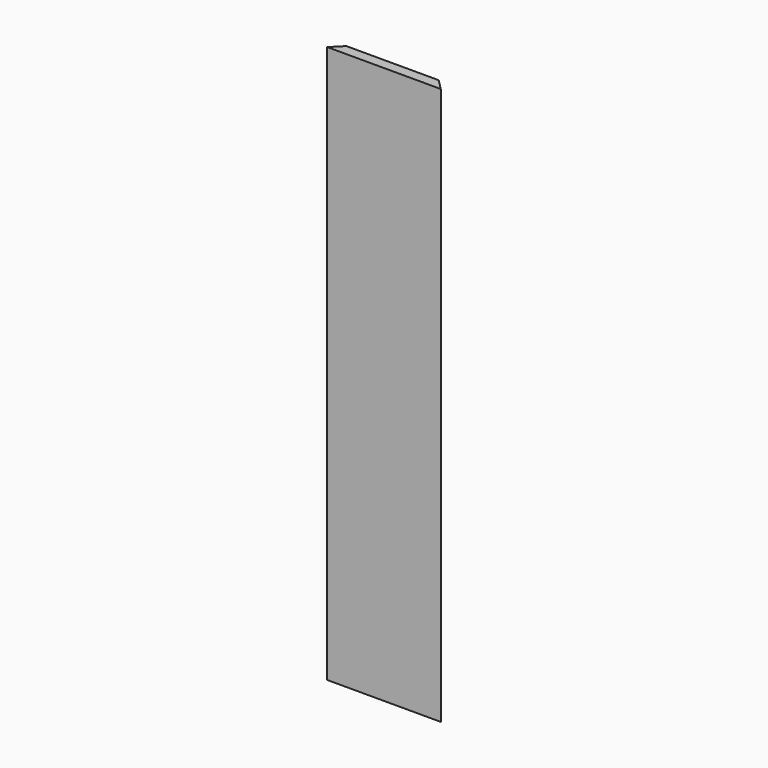
from build123d import *

# Parameters (mm, degrees)
F0_W     = 203.2
F0_H     = 996.95
F1_DEPTH = 19.05
F2_SIZE2 = 19.04999
F2_SIZE  = 19.04999


# Not quite as in the source:
# - a fillet or chamfer is up to 0.001 mm smaller than in the source, because OpenCascade refuses the exact size


with BuildPart() as f1:
    # F0 (on Front) → F1 (new body)
    with BuildSketch(Plane.XZ):
        with Locations((0, -22.3263513706)):
            Rectangle(F0_W, F0_H)
    extrude(amount=F1_DEPTH)

    # F2 (size 19.05 and 19.05 in the source; OpenCascade refuses exactly that, so slightly less here)
    f2_edges = [f1.edges().sort_by_distance(p)[0] for p in [
        (-101.6, 0, -22.326351),
        (101.6, 0, -22.326351),
    ]]
    chamfer(f2_edges, length=F2_SIZE, length2=F2_SIZE2)


solid = f1.part
